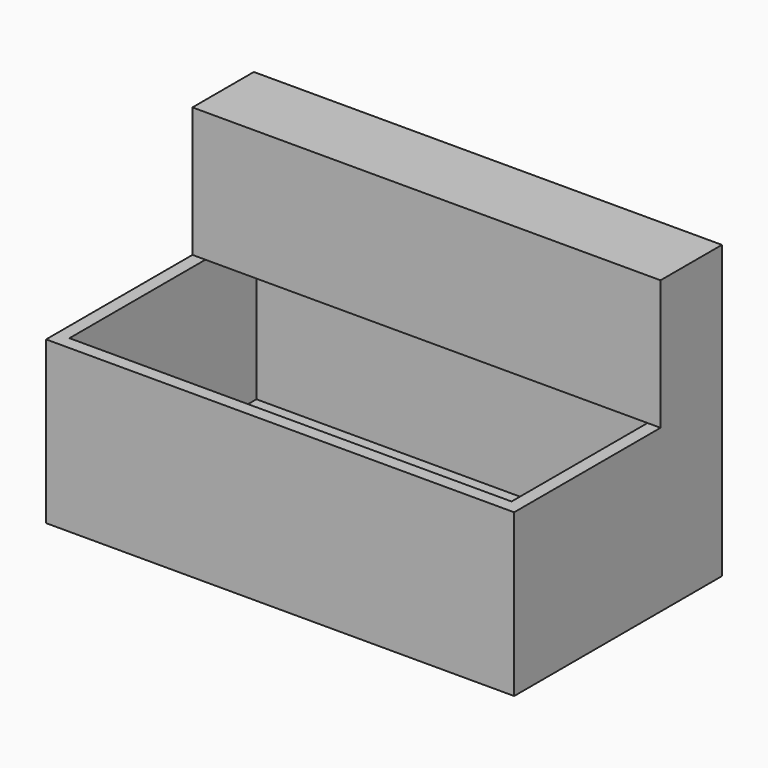
from build123d import *

# Parameters (mm, degrees)
F0_W     = 109.3384288251
F0_H     = 31.6438265145
F1_DEPTH = 50.8
F2_W     = 109.3384288251
F2_H     = 15.0109836832
F3_DEPTH = 25.4
F4_DEPTH = 17.78
F5_T     = -2.54


# Not quite as in the source:
# - a shell that OpenCascade refuses in one call is made with other operations: the cavity is built on its own and cut out


with BuildPart() as f1:
    # F0 (on Front) → F1 (new body)
    with BuildSketch(Plane.XZ):
        with Locations((2.1867696196, 0.8977539837)):
            Rectangle(F0_W, F0_H)
    extrude(amount=F1_DEPTH)

    # F2 (on face) → F3 (join)
    with BuildSketch(Plane.XY.offset(16.719667241)):
        with Locations((2.1867696196, -7.5054918416)):
            Rectangle(F2_W, F2_H)
    extrude(amount=F3_DEPTH)

    # F4 (cut): a face of the model
    f4_faces = [f1.faces().sort_by_distance(p)[0] for p in [
        (56.8559840322, -21.9693633853, 6.3658182119),
    ]]
    extrude(f4_faces, amount=-F4_DEPTH, mode=Mode.SUBTRACT)

    # F5: a shell. OpenCascade refuses it in one call, so the cavity is built on its own and cut out:
    # the body offset inwards by the wall thickness, plus a prism from it out through each open face.
    f5_core = offset(f1.part, amount=F5_T, kind=Kind.INTERSECTION, mode=Mode.PRIVATE)
    f5_exits = [f5_core.faces().sort_by_distance(p)[0] for p in [
        (-6.70323, -30.365492, 14.179667),
    ]]
    add(f5_core, mode=Mode.SUBTRACT)
    extrude(f5_exits, amount=-F5_T, mode=Mode.SUBTRACT)


solid = f1.part
